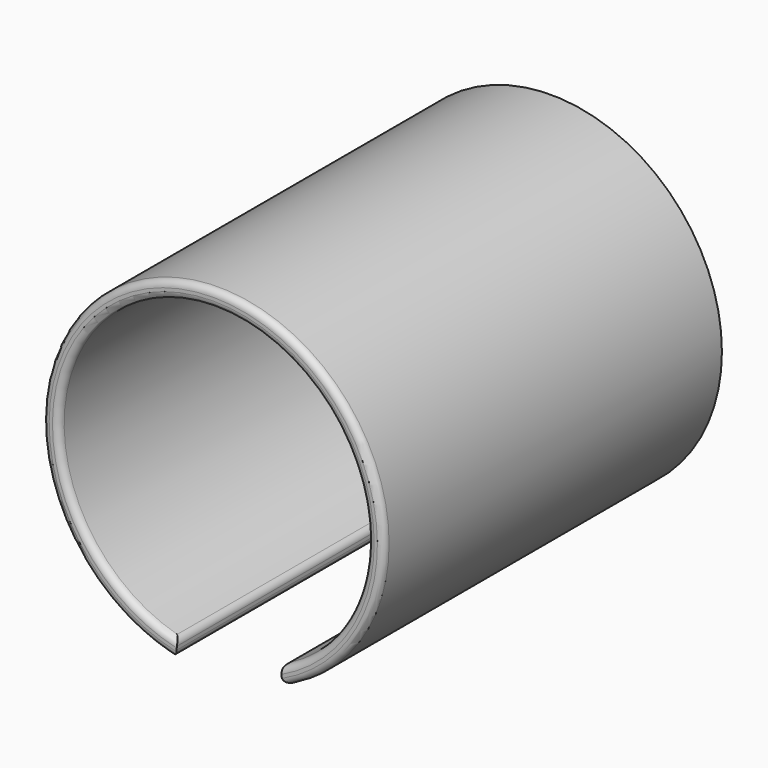
from build123d import *

# Parameters (mm, degrees)
F0_R      = 52.5
F1_DEPTH  = 130
F2_R      = 47.5
F3_DEPTH  = 125
F5_DEPTH  = 125
F6_R      = 2
F7_W      = 2.493188018
F7_H      = 93.4330150485
F8_DEPTH  = 1.5
F9_R      = 1
F10_W     = 45.0817196397
F10_H     = 2.4400168913
F11_DEPTH = 1.5
F12_R     = 0.99999
F13_W     = 44.996257755
F13_H     = 2.44
F14_DEPTH = 1.5
F15_R     = 0.99999


# Not quite as in the source:
# - a fillet or chamfer is up to 0.001 mm smaller than in the source, because OpenCascade refuses the exact size


with BuildPart() as f1:
    # F0 (on Front) → F1 (new body)
    with BuildSketch(Plane.XZ):
        Circle(F0_R)
    extrude(amount=-F1_DEPTH)

    # F2 (on face) → F3 (cut)
    with BuildSketch(Plane.XZ):
        Circle(F2_R)
    extrude(amount=-F3_DEPTH, mode=Mode.SUBTRACT)

    # F4 (on face) → F5 (cut)
    with BuildSketch(Plane.XZ):
        with BuildLine():
            ThreePointArc((20.9507066756, -42.6300116091), (5.1584797983, -47.2190648591), (-11.2520875409, -46.1480284083))
            Line((-11.2520875409, -46.1480284083), (-11.2520875409, -51.280020729))
            ThreePointArc((-11.2520875409, -51.280020729), (5.0973568866, -52.2519564492), (20.9507066756, -48.1385281224))
            Line((20.9507066756, -48.1385281224), (20.9507066756, -42.6300116091))
        make_face()
    extrude(amount=-F5_DEPTH, mode=Mode.SUBTRACT)

    # F6
    f6_edges = [f1.edges().sort_by_distance(p)[0] for p in [
        (-32.905284, 0, 40.90834),
        (-5.15848, 0, 47.219065),
        (-11.252088, 62.5, -46.148028),
        (20.950707, 62.5, -42.630012),
        (-11.252088, 62.5, -51.280021),
        (20.950707, 62.5, -48.138528),
    ]]
    fillet(f6_edges, radius=F6_R)

    # F7 (on face) → F8 (join)
    with BuildSketch(Plane.XZ.offset(-125)):
        Rectangle(F7_W, F7_H)
    extrude(amount=F8_DEPTH)

    # F9
    f9_edges = [f1.edges().sort_by_distance(p)[0] for p in [
        (-1.246594, 123.5, 0),
        (1.246594, 123.5, 0),
        (0, 123.5, 46.716508),
        (0, 123.5, -46.716508),
    ]]
    fillet(f9_edges, radius=F9_R)

    # F10 (on face) → F11 (join)
    with BuildSketch(Plane.XZ.offset(-125)):
        with Locations((-23.7874538288, -0.268576463)):
            Rectangle(F10_W, F10_H)
    extrude(amount=F11_DEPTH)

    # F12 (radius 1 in the source; OpenCascade refuses exactly that, so slightly less here)
    f12_edges = [f1.edges().sort_by_distance(p)[0] for p in [
        (-23.787454, 123.5, -1.488585),
        (-23.787454, 123.5, 0.951432),
        (-46.328314, 123.5, -0.268576),
        (-1.246594, 123.5, -0.268576),
    ]]
    fillet(f12_edges, radius=F12_R)

    # F13 (on face) → F14 (join)
    with BuildSketch(Plane.XZ.offset(-125)):
        with Locations((23.7447228865, -0.311423186)):
            Rectangle(F13_W, F13_H)
    extrude(amount=F14_DEPTH)

    # F15 (radius 1 in the source; OpenCascade refuses exactly that, so slightly less here)
    f15_edges = [f1.edges().sort_by_distance(p)[0] for p in [
        (23.744723, 123.5, 0.908577),
        (23.744723, 123.5, -1.531423),
        (1.246594, 123.5, -0.311423),
        (46.242852, 123.5, -0.311423),
    ]]
    fillet(f15_edges, radius=F15_R)


solid = f1.part
